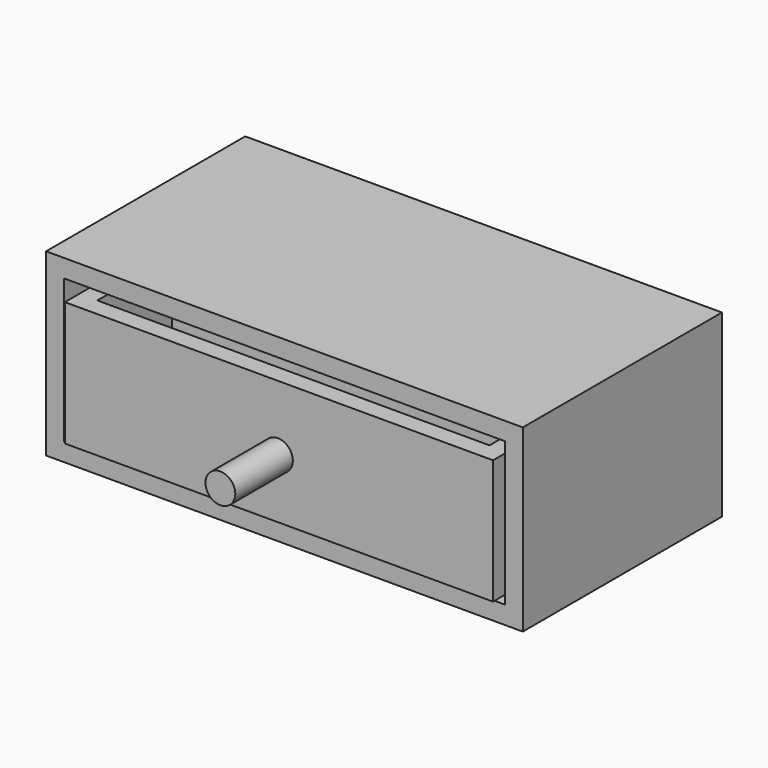
from build123d import *

# Parameters (mm, degrees)
F0_W     = 66.2849135697
F0_H     = 34.6089396626
F1_DEPTH = 25
F2_T     = -2.5
F3_W     = 59.5391076058
F3_H     = 17.3044716939
F4_DEPTH = 18
F5_T     = -2.5
F6_R     = 2.0739167643
F7_DEPTH = 10


# Not quite as in the source:
# - the program builds the solid bodies; features that only make, move or delete a surface that nothing else refers to are left out


with BuildPart() as f1:
    # F0 (on Top) → F1 (new body)
    with BuildSketch(Plane.XY):
        with Locations((-1.8626e-06, 0.4399446771)):
            Rectangle(F0_W, F0_H)
    extrude(amount=F1_DEPTH)

    # F2
    f2_openings = [f1.faces().sort_by_distance(p)[0] for p in [
        (-2e-06, -16.864525, 12.5),
    ]]
    offset(amount=F2_T, openings=f2_openings)


with BuildPart() as f4:
    # F3 (on Front) → F4 (new body)
    with BuildSketch(Plane.XZ):
        with Locations((0.1466469839, 11.7318448611)):
            Rectangle(F3_W, F3_H)
    extrude(amount=F4_DEPTH)

    # F5
    f5_openings = [f4.faces().sort_by_distance(p)[0] for p in [
        (0.146647, -9, 20.384081),
    ]]
    offset(amount=F5_T, openings=f5_openings)

    # F6 (on face) → F7 (join)
    with BuildSketch(Plane.XZ.offset(18)):
        with Locations((0, 11.2918997183)):
            Circle(F6_R)
    extrude(amount=F7_DEPTH)


solid = Compound([f1.part, f4.part])
